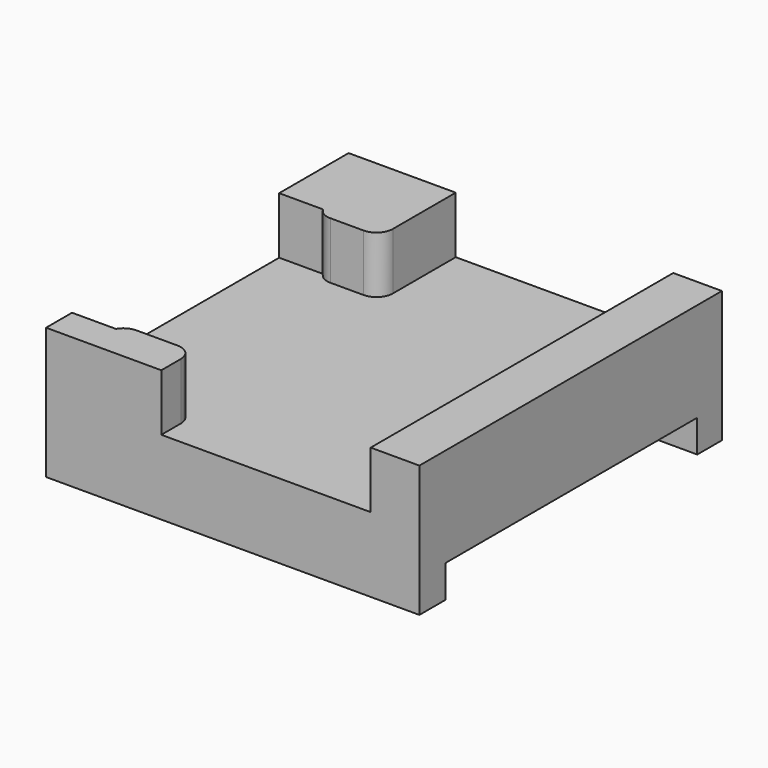
from build123d import *

# Parameters (mm, degrees)
F1_DEPTH    = 2.6
F0_W        = 3
F0_H        = 23.3
F0_W_2      = 4.4
F0_H_2      = 0.5
F0_W_3      = 3.9
F2_DEPTH    = 6.1
F3_T1_DEPTH = 6
F3_T3_DEPTH = 5.6650635095
F4_W        = 23
F4_H        = 2
F4_H_2      = 1.9
F5_DEPTH    = 2


# Not quite as in the source:
# - a fillet or chamfer that OpenCascade refuses, or shapes differently, is made with other operations: its cross-section is extruded or revolved along the edge and cut away or added


with BuildPart() as f1:
    # F0 (on Top) → F1 (new body)
    with BuildSketch(Plane.XY):
        Polygon((20, 0), (6.6, 0), (6.6, -5.35), (6.6, -5.85), (2.7, -5.85), (2.7, -5.35), (0, -5.35), (0, -21.3), (2.7, -21.3), (2.7, -20.8), (7.1, -20.8), (7.1, -21.3), (7.1, -23.3), (20, -23.3), align=None)
    extrude(amount=F1_DEPTH)

    # F0 (on Top) → F2 (join)
    with BuildSketch(Plane.XY):
        with Locations((21.5, -11.65)):
            Rectangle(F0_W, F0_H)
        Polygon((2.7, -21.3), (0, -21.3), (0, -23.3), (7.1, -23.3), (7.1, -21.3), align=None)
        Polygon((6.6, 0), (0, 0), (0, -5.35), (2.7, -5.35), (6.6, -5.35), align=None)
        with Locations((4.9, -21.05)):
            Rectangle(F0_W_2, F0_H_2)
        with Locations((4.65, -5.6)):
            Rectangle(F0_W_3, F0_H_2)
    extrude(amount=F2_DEPTH)

    # F3: fillet of radius 1 on 4 edges, made by hand

    # F3_s2 → F3_t1 (cut)
    with BuildSketch(Plane.XY.offset(2.6)):
        with BuildLine():
            ThreePointArc((7.1, -21.8), (6.8071067812, -21.0928932188), (6.1, -20.8))
            Line((6.1, -20.8), (7.1, -20.8))
            Line((7.1, -20.8), (7.1, -21.8))
        make_face()
        with BuildLine():
            ThreePointArc((5.6, -5.85), (6.3071067812, -5.5571067812), (6.6, -4.85))
            Line((6.6, -4.85), (6.6, -5.85))
            Line((6.6, -5.85), (5.6, -5.85))
        make_face()
    extrude(amount=F3_T1_DEPTH, mode=Mode.SUBTRACT)

    # F3_s4 → F3_t3 (cut)
    with BuildSketch(Plane.XY.offset(2.6)):
        with BuildLine():
            ThreePointArc((3.5660254038, -20.8), (3.0660254038, -20.9339745962), (2.7, -21.3))
            Line((2.7, -21.3), (2.7, -20.8))
            Line((2.7, -20.8), (3.5660254038, -20.8))
        make_face()
        with BuildLine():
            ThreePointArc((2.7, -5.35), (3.0660254038, -5.7160254038), (3.5660254038, -5.85))
            Line((3.5660254038, -5.85), (2.7, -5.85))
            Line((2.7, -5.85), (2.7, -5.35))
        make_face()
    extrude(amount=F3_T3_DEPTH, mode=Mode.SUBTRACT)

    # F4 (on Top) → F5 (join)
    with BuildSketch(Plane.XY):
        with Locations((11.5, -22.3)):
            Rectangle(F4_W, F4_H)
        with Locations((11.5, -0.95)):
            Rectangle(F4_W, F4_H_2)
    extrude(amount=-F5_DEPTH)


solid = f1.part
